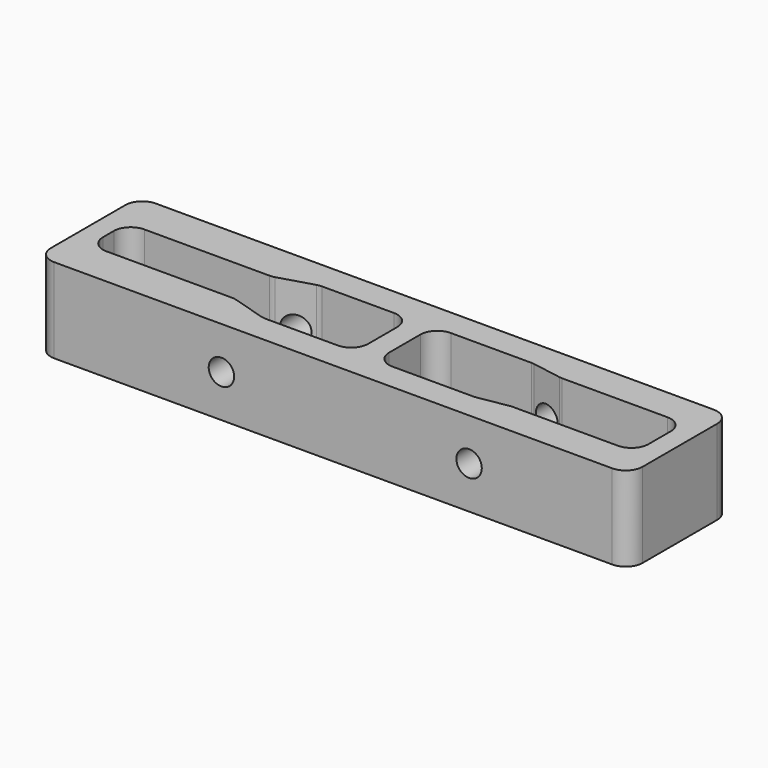
from build123d import *

# Parameters (mm, degrees)
F0_W     = 69.9
F0_H     = 15
F1_DEPTH = 5
F2_R     = 1.5
F3_DEPTH = 12.5
F4_R     = 2
F5_R     = 2


with BuildPart() as f1:
    # F0 (on Top) → F1 (new body, symmetric)
    with BuildSketch(Plane.XY):
        Rectangle(F0_W, F0_H)
        Polygon((-10.95, -4.15), (-15.45, -2.8), (-32.55, -2.8), (-32.55, 2.8), (-15.45, 2.8), (-10.95, 4.15), (-0.15, 4.15), (-0.15, -4.15), align=None, mode=Mode.SUBTRACT)
        Polygon((17.95, -3.65), (14.15, -4.3), (2.45, -4.3), (2.45, 4.3), (14.15, 4.3), (17.95, 3.65), (32.55, 3.65), (32.55, -3.65), align=None, mode=Mode.SUBTRACT)
    extrude(amount=F1_DEPTH, both=True)

    # F2 (on Front) → F3 (cut, symmetric)
    with BuildSketch(Plane.XZ):
        with Locations((-13.2, 0)):
            Circle(F2_R)
        with Locations((16.05, 0)):
            Circle(F2_R)
    extrude(amount=F3_DEPTH, both=True, mode=Mode.SUBTRACT)

    # F4
    f4_edges = [f1.edges().sort_by_distance(p)[0] for p in [
        (-34.95, 7.5, 0),
        (-34.95, -7.5, 0),
        (34.95, -7.5, 0),
        (34.95, 7.5, 0),
    ]]
    fillet(f4_edges, radius=F4_R)

    # F5
    f5_edges = [f1.edges().sort_by_distance(p)[0] for p in [
        (-32.55, 2.8, 0),
        (32.55, 3.65, 0),
        (32.55, -3.65, 0),
        (-32.55, -2.8, 0),
        (-15.45, 2.8, 0),
        (-10.95, 4.15, 0),
        (14.15, 4.3, 0),
        (17.95, 3.65, 0),
        (-15.45, -2.8, 0),
        (-10.95, -4.15, 0),
        (14.15, -4.3, 0),
        (17.95, -3.65, 0),
        (-0.15, 4.15, 0),
        (-0.15, -4.15, 0),
        (2.45, -4.3, 0),
        (2.45, 4.3, 0),
    ]]
    fillet(f5_edges, radius=F5_R)


solid = f1.part
